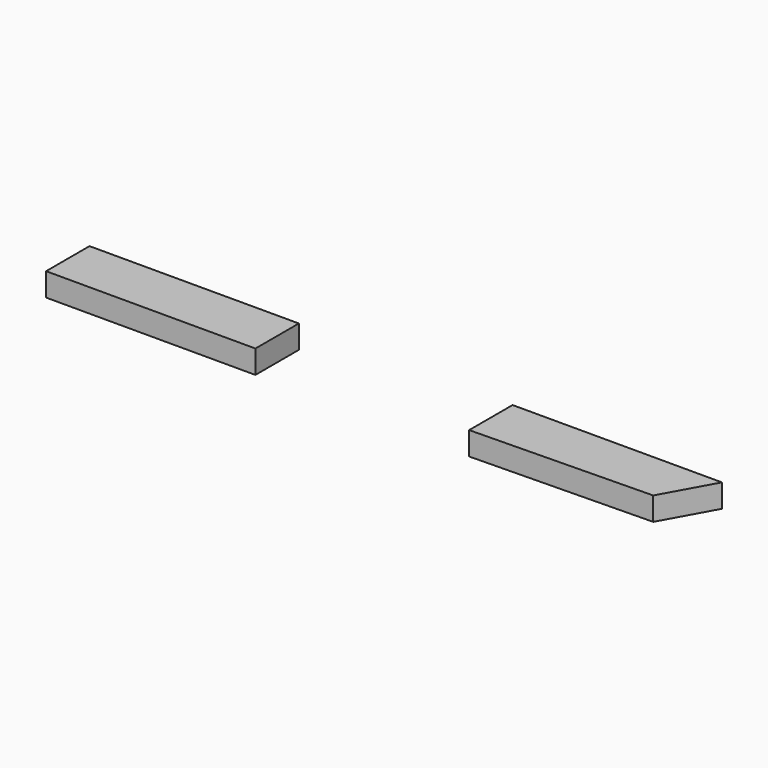
from build123d import *

# Parameters (mm, degrees)
F1_DEPTH = 19.05
F0_W     = 342.9
F0_H     = 88.9
F2_DEPTH = 19.05


# Not quite as in the source:
# - a feature names something its author has since deleted; it is built from what else it names


with BuildPart() as f1:
    # F0 (on Top) → F1 (new body, symmetric)
    with BuildSketch(Plane.XY):
        Polygon((-296.9577699824, -5.6861853861), (0, 0), (45.9422300176, 83.2138146139), (-296.9577699824, 83.2138146139), align=None)
    extrude(amount=F1_DEPTH, both=True)


with BuildPart() as f2:
    # F0 (on Top) → F2 (new body, symmetric)
    with BuildSketch(Plane.XY):
        with Locations((-823.031742382, 44.45)):
            Rectangle(F0_W, F0_H)
    extrude(amount=F2_DEPTH, both=True)


solid = Compound([f1.part, f2.part])
